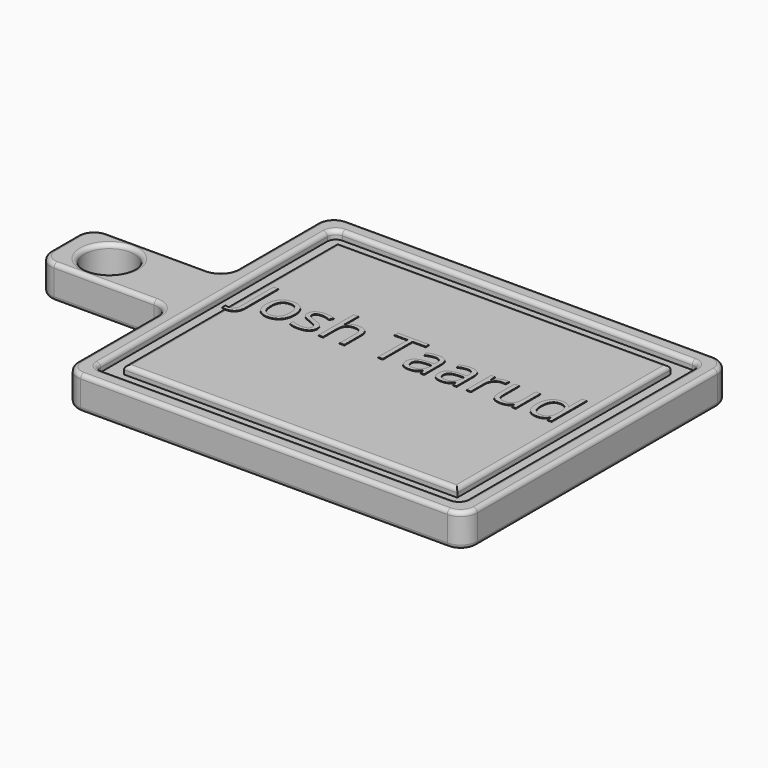
from build123d import *

# Parameters (mm, degrees)
F0_W         = 101.6
F0_H         = 50.8
F1_DEPTH     = 25.4
F2_R         = 19.05
F3_DEPTH     = 25.4
F5_DEPTH     = 6.35
F6_R         = 6.35
F7_R         = 12.7
F8_R         = 3.17499
F9_TEXT_SIZE = 44.3891766313
F10_DEPTH    = 0.508


# Not quite as in the source:
# - a fillet or chamfer is up to 0.001 mm smaller than in the source, because OpenCascade refuses the exact size
# - Text() gives the source's letters only with a copy of the font that has no kerning and outlines rounded to 1/6400 em; it was checked with that copy


with BuildPart() as f1:
    # F0 (on Top) → F1 (new body)
    with BuildSketch(Plane.XY):
        Polygon((0, 101.6), (0, 0), (304.8, 0), (304.8, 254), (0, 254), (0, 152.4), align=None)
        with Locations((-50.8, 127)):
            Rectangle(F0_W, F0_H)
    extrude(amount=F1_DEPTH)

    # F2 (on Top) → F3 (cut)
    with BuildSketch(Plane.XY):
        with Locations((-67.1032518148, 127)):
            Circle(F2_R)
    extrude(amount=F3_DEPTH, mode=Mode.SUBTRACT)

    # F4 (on face) → F5 (cut)
    with BuildSketch(Plane.XY.offset(25.4)):
        Polygon((12.6999982595, 101.6), (12.6999982595, 12.6999982595), (292.1000017405, 12.6999982595), (292.1000017405, 241.3000017405), (12.6999982595, 241.3000017405), (12.6999982595, 152.4), align=None)
        Polygon((25.4000046253, 101.6), (25.4000046253, 152.4), (25.4000046253, 228.5999953747), (279.3999953747, 228.5999953747), (279.3999953747, 25.4000046253), (25.4000046253, 25.4000046253), align=None, mode=Mode.SUBTRACT)
    extrude(amount=-F5_DEPTH, mode=Mode.SUBTRACT)

    # F6
    f6_edges = [f1.edges().sort_by_distance(p)[0] for p in [
        (12.699998, 241.300002, 22.225),
        (292.100002, 241.300002, 22.225),
        (12.699998, 12.699998, 22.225),
        (292.100002, 12.699998, 22.225),
    ]]
    fillet(f6_edges, radius=F6_R)

    # F7
    f7_edges = [f1.edges().sort_by_distance(p)[0] for p in [
        (0, 254, 12.7),
        (-101.6, 152.4, 12.7),
        (-101.6, 101.6, 12.7),
        (0, 0, 12.7),
        (304.8, 254, 12.7),
        (304.8, 0, 12.7),
        (0, 152.4, 12.7),
        (0, 101.6, 12.7),
    ]]
    fillet(f7_edges, radius=F7_R)

    # F8 (radius 3.175 in the source; OpenCascade refuses exactly that, so slightly less here)
    f8_edges = [f1.edges().sort_by_distance(p)[0] for p in [
        (152.4, 228.599995, 25.4),
        (279.399995, 127, 25.4),
        (152.4, 25.400005, 25.4),
        (25.400005, 127, 25.4),
        (0, 50.8, 25.4),
        (-3.719744, 97.880256, 25.4),
        (3.719744, 3.719744, 25.4),
        (-50.8, 101.6, 25.4),
        (152.4, 0, 25.4),
        (-97.880256, 105.319744, 25.4),
        (301.080256, 3.719744, 25.4),
        (-101.6, 127, 25.4),
        (304.8, 127, 25.4),
        (-97.880256, 148.680256, 25.4),
        (301.080256, 250.280256, 25.4),
        (-50.8, 152.4, 25.4),
        (152.4, 254, 25.4),
        (-3.719744, 156.119744, 25.4),
        (3.719744, 250.280256, 25.4),
        (0, 203.2, 25.4),
        (152.4, 12.699998, 25.4),
        (14.55987, 14.55987, 25.4),
        (290.24013, 14.55987, 25.4),
        (12.699998, 127, 25.4),
        (292.100002, 127, 25.4),
        (14.55987, 239.44013, 25.4),
        (290.24013, 239.44013, 25.4),
        (152.4, 241.300002, 25.4),
        (-86.153252, 127, 25.4),
        (0, 50.8, 0),
        (-3.719744, 97.880256, 0),
        (3.719744, 3.719744, 0),
        (-50.8, 101.6, 0),
        (152.4, 0, 0),
        (-97.880256, 105.319744, 0),
        (301.080256, 3.719744, 0),
        (-101.6, 127, 0),
        (304.8, 127, 0),
        (-97.880256, 148.680256, 0),
        (301.080256, 250.280256, 0),
        (-50.8, 152.4, 0),
        (152.4, 254, 0),
        (-3.719744, 156.119744, 0),
        (3.719744, 250.280256, 0),
        (0, 203.2, 0),
        (-86.153252, 127, 0),
    ]]
    fillet(f8_edges, radius=F8_R)

    # F9 (on face) → F10 (join)
    with BuildSketch(Plane.XY.offset(25.4)):
        with Locations((28.5750046253, 127)):
            Text('Josh Taarud', F9_TEXT_SIZE, font='Open Sans', text_align=(TextAlign.LEFT, TextAlign.BOTTOM))
    extrude(amount=F10_DEPTH)


solid = f1.part
